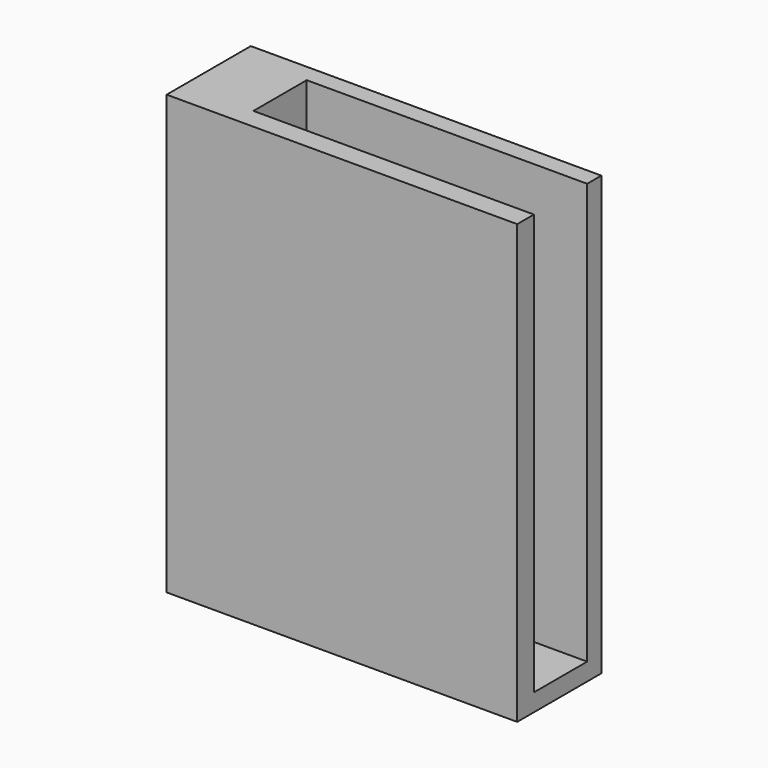
from build123d import *

# Parameters (mm, degrees)
F0_W     = 10
F0_H     = 12.5
F1_DEPTH = 3
F2_W     = 1.9
F2_H     = 12
F3_DEPTH = 8


# Not quite as in the source:
# - a feature names something its author has since deleted; it is built from what else it names


with BuildPart() as f1:
    # F0 (on Front) → F1 (new body)
    with BuildSketch(Plane.XZ):
        with Locations((5, 6.25)):
            Rectangle(F0_W, F0_H)
    extrude(amount=F1_DEPTH)

    # F2 (on face) → F3 (cut)
    with BuildSketch(Plane.YZ.offset(10)):
        with Locations((-1.4556478869, 6.5)):
            Rectangle(F2_W, F2_H)
    extrude(amount=-F3_DEPTH, mode=Mode.SUBTRACT)


solid = f1.part
